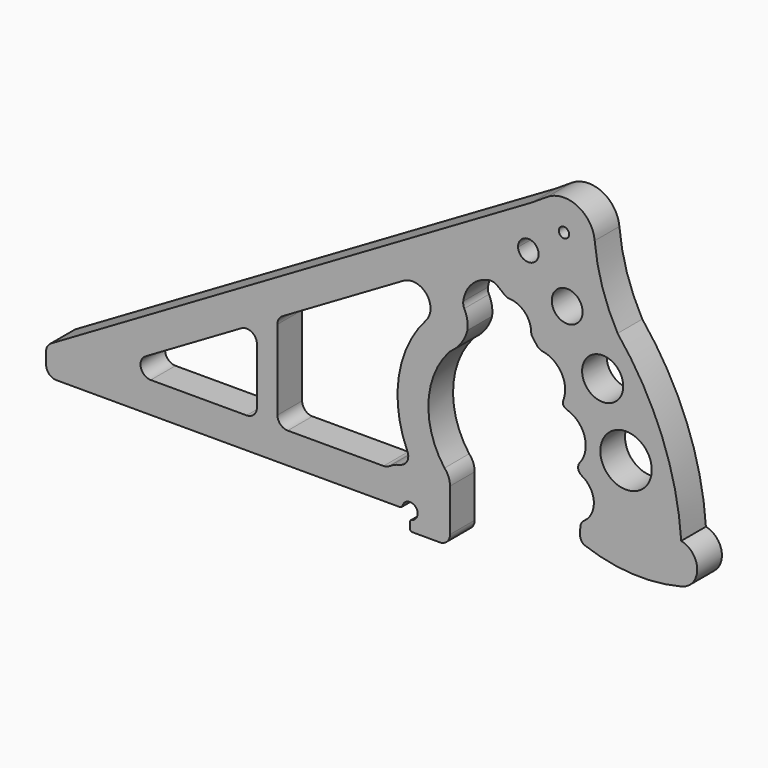
from build123d import *

# Parameters (mm, degrees)
F1_DEPTH    = 19.05
F2_R        = 3.175
F2_R_2      = 9.525
F2_R_3      = 12.7
F2_R_4      = 15.875
F3_DEPTH    = 25.4
F5_DEPTH    = 25.4
F6_T1_DEPTH = 30.0603271211
F6_T3_DEPTH = 31.1986000008
F6_T5_DEPTH = 28.3963352446
F6_T7_DEPTH = 32.4334586234


# Not quite as in the source:
# - a fillet or chamfer that OpenCascade refuses, or shapes differently, is made with other operations: its cross-section is extruded or revolved along the edge and cut away or added


with BuildPart() as f1:
    # F0 (on Front) → F1 (new body)
    with BuildSketch(Plane.XZ):
        with BuildLine():
            ThreePointArc((-97.6744983316, -31.75), (-95.8146263921, -36.2401280605), (-91.3244983316, -38.1))
            Line((-91.3244983316, -38.1), (120.8516389379, -38.1))
            ThreePointArc((120.8516389379, -38.1), (121.8237801796, -37.7675289464), (122.3887292034, -36.909375))
            ThreePointArc((122.3887292034, -36.909375), (130.3675960454, -34.7324039546), (128.190625, -42.7112707966))
            ThreePointArc((128.190625, -42.7112707966), (127.3324710536, -43.2762198204), (127, -44.2483610621))
            Line((127, -44.2483610621), (127, -47.6885))
            ThreePointArc((127, -47.6885), (127.4649679849, -48.8110320151), (128.5875, -49.276))
            Line((128.5875, -49.276), (145.4092243424, -49.276))
            ThreePointArc((145.4092243424, -49.276), (149.8993524029, -47.4161280605), (151.7592243424, -42.926))
            Line((151.7592243424, -42.926), (151.7592243424, -16.6167677244))
            ThreePointArc((151.7592243424, -16.6167677244), (150.8744160327, -11.9593816205), (148.3432801973, -7.95095519))
            ThreePointArc((148.3432801973, -7.95095519), (138.4290547294, 24.5532823111), (151.2244431733, 56.0349493051))
            ThreePointArc((151.2244431733, 56.0349493051), (151.7400284969, 56.5513745002), (152.3114587754, 57.0052364228))
            ThreePointArc((152.3114587754, 57.0052364228), (158.6954603174, 63.4018980936), (162.5374758377, 71.5818536535))
            ThreePointArc((162.5374758377, 71.5818536535), (162.3873847727, 77.3115690897), (160.5681351866, 82.7468701164))
            ThreePointArc((160.5681351866, 82.7468701164), (159.9697528023, 84.5410858194), (159.9263668127, 86.4319557574))
            ThreePointArc((159.9263668127, 86.4319557574), (165.1411573537, 97.4071817121), (175.8442055157, 103.1599536687))
            ThreePointArc((175.8442055157, 103.1599536687), (178.4583890799, 103.0782041484), (180.8178773791, 101.9497301092))
            ThreePointArc((180.8178773791, 101.9497301092), (221.6873319491, 49.6461946462), (231.9580536588, -15.9318841175))
            ThreePointArc((231.9580536588, -15.9318841175), (232.4585750307, -19.0998901862), (234.443503066, -21.6191846886))
            ThreePointArc((234.443503066, -21.6191846886), (264.2459103293, -27.7561805118), (294.5264875889, -24.767395266))
            ThreePointArc((294.5264875889, -24.767395266), (304.4097460434, -12.383697633), (294.5264875889, 0))
            ThreePointArc((294.5264875889, 0), (282.6289913598, 53.0536935026), (255.2546977003, 100.031271744))
            ThreePointArc((255.2546977003, 100.031271744), (245.7643329114, 122.1712128334), (241.0873952711, 145.8010725364))
            ThreePointArc((241.0873952711, 145.8010725364), (230.45685595, 161.2038903493), (211.7757176902, 160.0768428105))
            Line((211.7757176902, 160.0768428105), (202.1868032782, 153.8799835291))
            Line((202.1868032782, 153.8799835291), (-94.5235117526, -19.159885704))
            ThreePointArc((-94.5235117526, -19.159885704), (-96.8306873596, -21.4822422795), (-97.6744983316, -24.6452127802))
            Line((-97.6744983316, -24.6452127802), (-97.6744983316, -31.75))
        make_face()
    extrude(amount=F1_DEPTH)

    # F2 (on face) → F3 (cut)
    with BuildSketch(Plane.XZ.offset(19.05)):
        with Locations((222.1155585436, 144.0771493407)):
            Circle(F2_R)
        with BuildLine():
            Line((203.4512059186, 132.5644525933), (193.776246746, 126.9220681353))
            ThreePointArc((193.776246746, 126.9220681353), (200.2394873385, 120.8083090531), (206.4718912023, 127.1572200738))
            ThreePointArc((206.4718912023, 127.1572200738), (205.6655203588, 130.254101695), (203.4512059186, 132.5644525933))
        make_face()
        with BuildLine():
            ThreePointArc((203.4512059186, 132.5644525933), (196.9228777813, 132.6425471499), (193.776246746, 126.9220681353))
            Line((193.776246746, 126.9220681353), (203.4512059186, 132.5644525933))
        make_face()
        with Locations((224.0934852203, 104.6425497844)):
            Circle(F2_R_2)
        with Locations((246.0011737906, 72.412781237)):
            Circle(F2_R_3)
        with Locations((260.4474416869, 32.6195944174)):
            Circle(F2_R_4)
        with BuildLine():
            ThreePointArc((-36.2271326674, -7.2146729239), (-39.1581407363, -14.3569057105), (-33.0281192464, -19.05))
            Line((-33.0281192464, -19.05), (26.1524232063, -19.05))
            ThreePointArc((26.1524232063, -19.05), (30.6425512669, -17.1901280605), (32.5024232063, -12.7))
            Line((32.5024232063, -12.7), (32.5024232063, 21.8137759235))
            ThreePointArc((32.5024232063, 21.8137759235), (29.315393707, 27.3199649515), (22.9534097853, 27.2991029996))
            Line((22.9534097853, 27.2991029996), (-36.2271326674, -7.2146729239))
        make_face()
        with BuildLine():
            ThreePointArc((125.4190243086, -6.2600999334), (120.1455601031, 32.9262812272), (136.9919967338, 68.6974912436))
            ThreePointArc((136.9919967338, 68.6974912436), (137.1991099249, 83.0744541178), (123.0586985781, 85.6799721664))
            Line((123.0586985781, 85.6799721664), (48.3534097853, 42.1122471873))
            ThreePointArc((48.3534097853, 42.1122471873), (46.0462341784, 39.7898906118), (45.2024232063, 36.6269201112))
            Line((45.2024232063, 36.6269201112), (45.2024232063, 36.5713226157))
            Line((45.2024232063, 36.5713226157), (45.2024232063, -12.7))
            ThreePointArc((45.2024232063, -12.7), (47.0622951458, -17.1901280605), (51.5524232063, -19.05))
            Line((51.5524232063, -19.05), (110.732965659, -19.05))
            ThreePointArc((110.732965659, -19.05), (112.5171616301, -18.7941894241), (114.1576044677, -18.0473684211))
            ThreePointArc((114.1576044677, -18.0473684211), (117.5440512909, -16.2454766636), (121.1758845472, -15.0107203351))
            ThreePointArc((121.1758845472, -15.0107203351), (125.336500367, -11.6241351048), (125.4190243086, -6.2600999334))
        make_face()
    extrude(amount=-F3_DEPTH, mode=Mode.SUBTRACT)

    # F4 (on face) → F5 (cut)
    with BuildSketch(Plane.XZ.offset(19.05)):
        with BuildLine():
            Line((205.7570372824, 42.3802169454), (212.9491877633, 45.8553555323))
            ThreePointArc((212.9491877633, 45.8553555323), (212.5656514739, 46.730082771), (212.1753107443, 47.6017948463))
            ThreePointArc((212.1753107443, 47.6017948463), (208.6337520482, 45.3996132397), (205.7570372824, 42.3802169454))
        make_face()
        with BuildLine():
            ThreePointArc((212.1753107443, 47.6017948463), (212.5656514739, 46.730082771), (212.9491877633, 45.8553555323))
            Line((212.9491877633, 45.8553555323), (205.7570372824, 42.3802169454))
            ThreePointArc((205.7570372824, 42.3802169454), (213.5341104331, 44.0137836863), (219.6469644258, 49.09162015))
            ThreePointArc((219.6469644258, 49.09162015), (215.8240199222, 48.7836130904), (212.1753107443, 47.6017948463))
        make_face()
        with BuildLine():
            ThreePointArc((205.7570372824, 42.3802169454), (208.6337520482, 45.3996132397), (212.1753107443, 47.6017948463))
            ThreePointArc((212.1753107443, 47.6017948463), (205.3746994644, 60.5221639094), (197.0859881764, 72.5422103192))
            Line((197.0859881764, 72.5422103192), (193.6454970545, 69.4190230989))
            ThreePointArc((193.6454970545, 69.4190230989), (191.2850857199, 52.1297449914), (205.7570372824, 42.3802169454))
        make_face()
        with BuildLine():
            ThreePointArc((197.0859881764, 72.5422103192), (205.3746994644, 60.5221639094), (212.1753107443, 47.6017948463))
            ThreePointArc((212.1753107443, 47.6017948463), (215.8240199222, 48.7836130904), (219.6469644258, 49.09162015))
            ThreePointArc((219.6469644258, 49.09162015), (222.0367215402, 53.7280102211), (222.8607258742, 58.8785508543))
            ThreePointArc((222.8607258742, 58.8785508543), (214.0841075429, 73.4647831759), (197.0859881764, 72.5422103192))
        make_face()
        with BuildLine():
            ThreePointArc((219.6469644258, 49.09162015), (213.5341104331, 44.0137836863), (205.7570372824, 42.3802169454))
            ThreePointArc((205.7570372824, 42.3802169454), (205.0900299154, 23.784029323), (222.1616065465, 16.3796816648))
            ThreePointArc((222.1616065465, 16.3796816648), (223.0725498981, 16.6422099505), (223.9991050166, 16.8427953515))
            ThreePointArc((223.9991050166, 16.8427953515), (232.3605019958, 22.823896366), (235.5613691058, 32.5932862411))
            ThreePointArc((235.5613691058, 32.5932862411), (230.9343591767, 44.0547793603), (219.6469644258, 49.09162015))
        make_face()
        with BuildLine():
            ThreePointArc((195.5812538731, 71.3904075622), (196.3170814503, 71.9879165163), (197.0859881764, 72.5422103192))
            ThreePointArc((197.0859881764, 72.5422103192), (187.8014437334, 83.1128874452), (177.3667262781, 92.5499766177))
            ThreePointArc((177.3667262781, 92.5499766177), (177.1387060987, 73.9342161605), (195.5812538731, 71.3904075622))
        make_face()
        with BuildLine():
            ThreePointArc((177.3667262781, 92.5499766177), (187.8014437334, 83.1128874452), (197.0859881764, 72.5422103192))
            ThreePointArc((197.0859881764, 72.5422103192), (200.6187749377, 77.3113358236), (201.8706292258, 83.1128874452))
            ThreePointArc((201.8706292258, 83.1128874452), (192.8578260854, 96.2420526102), (177.3667262781, 92.5499766177))
        make_face()
        with BuildLine():
            Line((193.6454970545, 69.4190230989), (197.0859881764, 72.5422103192))
            ThreePointArc((197.0859881764, 72.5422103192), (196.3530349145, 71.9409463118), (195.5812538731, 71.3904075622))
            ThreePointArc((195.5812538731, 71.3904075622), (194.5720627472, 70.4452814273), (193.6454970545, 69.4190230989))
        make_face()
        with BuildLine():
            ThreePointArc((195.5812538731, 71.3904075622), (196.3530349145, 71.9409463118), (197.0859881764, 72.5422103192))
            ThreePointArc((197.0859881764, 72.5422103192), (196.3170814503, 71.9879165163), (195.5812538731, 71.3904075622))
        make_face()
        with BuildLine():
            ThreePointArc((223.9991050166, 16.8427953515), (223.0725498981, 16.6422099505), (222.1616065465, 16.3796816648))
            ThreePointArc((222.1616065465, 16.3796816648), (223.0870059682, 16.5848525296), (223.9991050166, 16.8427953515))
        make_face()
        with BuildLine():
            ThreePointArc((223.9991050166, 16.8427953515), (223.0870059682, 16.5848525296), (222.1616065465, 16.3796816648))
            ThreePointArc((222.1616065465, 16.3796816648), (218.2420246677, -8.38309145), (240.5801356684, 2.9996521278))
            ThreePointArc((240.5801356684, 2.9996521278), (235.5276670104, 13.7996890697), (223.9991050166, 16.8427953515))
        make_face()
    extrude(amount=-F5_DEPTH, mode=Mode.SUBTRACT)

    # F6: fillet of radius 5.08 on 8 edges, made by hand

    # F6_s2 → F6_t1 (cut)
    with BuildSketch(Plane.XZ.offset(-5.5051635606)):
        with BuildLine():
            ThreePointArc((221.8713115401, 49.2200601176), (221.4599286068, 51.1151221825), (221.7886262098, 53.0262616419))
            ThreePointArc((221.7886262098, 53.0262616419), (221.4135293391, 52.1191653521), (220.9851854038, 51.2359650268))
            ThreePointArc((220.9851854038, 51.2359650268), (221.432449207, 50.2298590785), (221.8713115401, 49.2200601176))
        make_face()
        with BuildLine():
            ThreePointArc((208.8420945961, 75.1986750012), (207.0161625579, 75.8517204357), (205.5679730948, 77.1413883878))
            ThreePointArc((205.5679730948, 77.1413883878), (206.2316951899, 76.2628856448), (206.8880718736, 75.3788812682))
            ThreePointArc((206.8880718736, 75.3788812682), (207.8677630854, 75.3178364408), (208.8420945961, 75.1986750012))
        make_face()
    extrude(amount=F6_T1_DEPTH, mode=Mode.SUBTRACT)

    # F6_s4 → F6_t3 (cut)
    with BuildSketch(Plane.XZ.offset(-6.0743000004)):
        with BuildLine():
            ThreePointArc((224.1373418719, 48.2996925298), (222.3088529855, 49.3521578516), (221.0656189971, 51.0566883182))
            ThreePointArc((221.0656189971, 51.0566883182), (221.5569923707, 49.9456220571), (222.0381267809, 48.830083753))
            ThreePointArc((222.0381267809, 48.830083753), (223.0964388832, 48.5993395729), (224.1373418719, 48.2996925298))
        make_face()
        with BuildLine():
            ThreePointArc((230.8865844012, 18.2789289832), (230.9876985591, 20.3862568619), (231.9362009526, 22.2707722029))
            ThreePointArc((231.9362009526, 22.2707722029), (231.2315639977, 21.4481215212), (230.4744978403, 20.6734485479))
            ThreePointArc((230.4744978403, 20.6734485479), (230.6860466781, 19.4771362484), (230.8865844012, 18.2789289832))
        make_face()
    extrude(amount=F6_T3_DEPTH, mode=Mode.SUBTRACT)

    # F6_s6 → F6_t5 (cut)
    with BuildSketch(Plane.XZ.offset(-4.6731676223)):
        with BuildLine():
            ThreePointArc((203.002520704, 80.4003376681), (202.1795489166, 81.8431560004), (201.8659860021, 83.4743168145))
            ThreePointArc((201.8659860021, 83.4743168145), (201.8632603647, 82.657592546), (201.8131477205, 81.8424025787))
            ThreePointArc((201.8131477205, 81.8424025787), (202.4103850279, 81.1234739617), (203.002520704, 80.4003376681))
        make_face()
        with BuildLine():
            ThreePointArc((188.3671023799, 97.170697044), (186.7406676624, 97.5079171684), (185.3099539983, 98.3517570313))
            ThreePointArc((185.3099539983, 98.3517570313), (186.0244140953, 97.749181287), (186.7345928658, 97.1415655599))
            ThreePointArc((186.7345928658, 97.1415655599), (187.5504246675, 97.1798334481), (188.3671023799, 97.170697044))
        make_face()
    extrude(amount=F6_T5_DEPTH, mode=Mode.SUBTRACT)

    # F6_s8 → F6_t7 (cut)
    with BuildSketch(Plane.XZ.offset(-6.6917293117)):
        with BuildLine():
            ThreePointArc((232.2568768174, -12.4388497815), (232.9187668001, -10.2742241066), (234.4552271906, -8.6119990526))
            ThreePointArc((234.4552271906, -8.6119990526), (233.4629344096, -9.2319420298), (232.4225614415, -9.767290837))
            ThreePointArc((232.4225614415, -9.767290837), (232.3464860605, -11.1034899805), (232.2568768174, -12.4388497815))
        make_face()
        with BuildLine():
            ThreePointArc((233.3303189509, 15.3056746343), (231.6446289063, 16.816353864), (230.7824945926, 18.9093008502))
            ThreePointArc((230.7824945926, 18.9093008502), (230.9970416723, 17.5882462846), (231.1981934117, 16.2650858285))
            ThreePointArc((231.1981934117, 16.2650858285), (232.284220259, 15.829746943), (233.3303189509, 15.3056746343))
        make_face()
    extrude(amount=F6_T7_DEPTH, mode=Mode.SUBTRACT)


solid = f1.part
